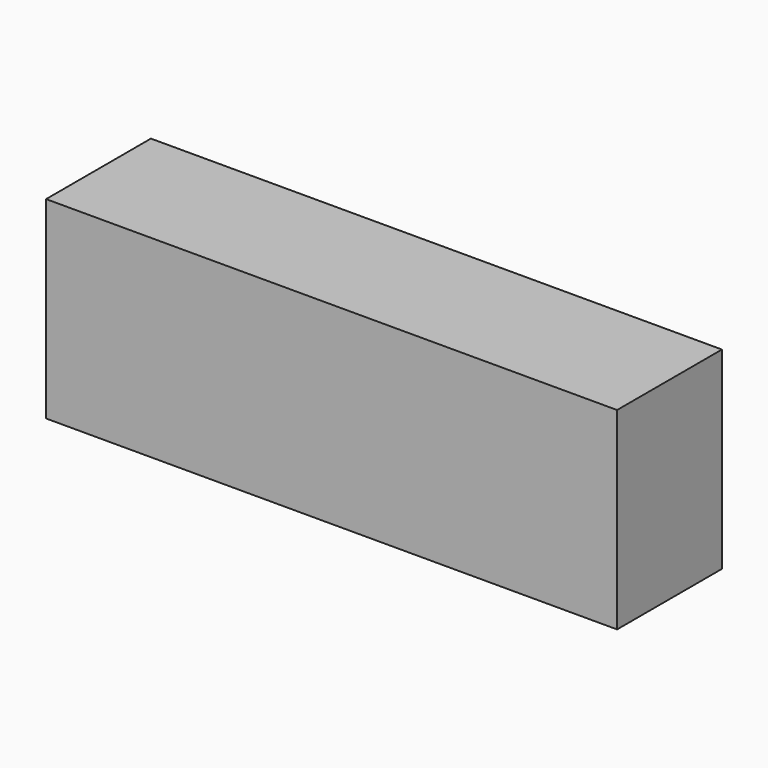
from build123d import *

# Parameters (mm, degrees)
F1_E0_W  = 110.6793768704
F1_E0_H  = 37.4396033585
F2_DEPTH = 25.4


with BuildPart() as f2:
    # F1_E0 (on explicit) → F2 (new body)
    with BuildSketch(Plane(origin=(60.3353269398, 47.594293952, 0), x_dir=(-1, 0, 0), z_dir=(0, 1, 0))):
        with Locations((55.3396884352, 18.7198016793)):
            Rectangle(F1_E0_W, F1_E0_H)
    extrude(amount=F2_DEPTH)


solid = f2.part
